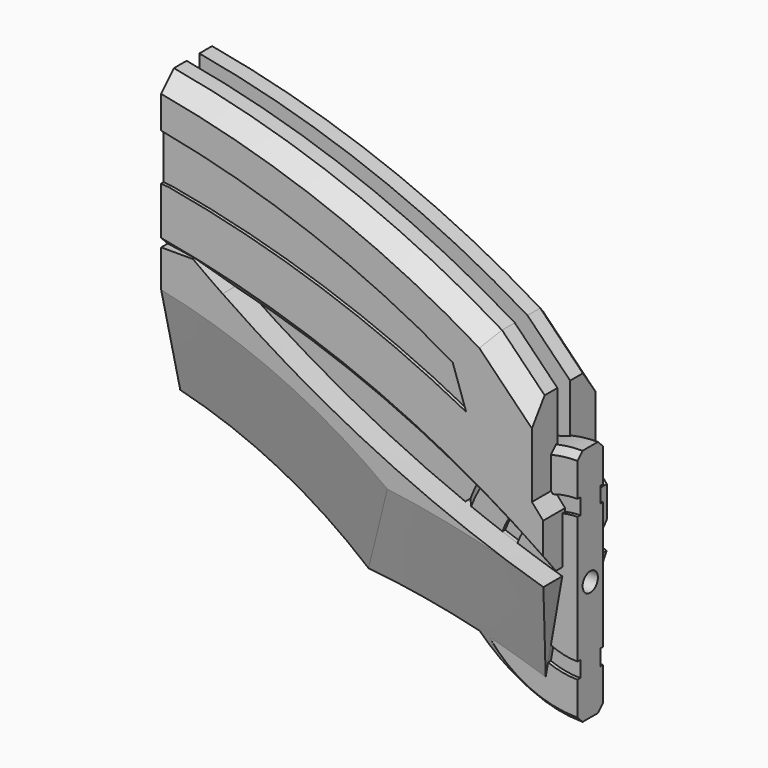
from build123d import *

# Parameters (mm, degrees)
F3_DEPTH     = 31.75
F5_DEPTH     = 6.35
F6_SIZE      = 12.7
F7_SIZE      = 12.7
F9_DEPTH     = 31.75
F11_DEPTH    = 12.7
F13_T2_ANGLE = 48.1784563201
F13_T4_ANGLE = 86.2150976381
F13_T6_ANGLE = 86.2150976381
F13_T8_ANGLE = 48.1784563201
F15_DEPTH    = 12.7
F16_SIZE     = 5.08
F18_DEPTH    = 2.54
F20_DEPTH    = 2.54
F21_R        = 7.62
F22_DEPTH    = 38.1
F24_DEPTH    = 2.794
F26_DEPTH    = 2.54
F27_R        = 10.16
F27_R_2      = 9.525
F28_DEPTH    = 76.2


# Not quite as in the source:
# - a fillet or chamfer that OpenCascade refuses, or shapes differently, is made with other operations: its cross-section is extruded or revolved along the edge and cut away or added
# - a feature of the source that left no trace in its solid (it failed there, or was rolled back) is left out
# - a feature names something its author has since deleted; it is built from what else it names


with BuildPart() as f3:
    # F2 (on Front) → F3 (new body, symmetric)
    with BuildSketch(Plane.XZ):
        with BuildLine():
            Line((37.9477068782, 57.15), (37.9477068782, -69.85))
            ThreePointArc((37.9477068782, -69.85), (197.3095607255, -116.6415507663), (342.7477068782, -196.85))
            Line((342.7477068782, -196.85), (342.7477068782, -156.4439684153))
            Line((342.7477068782, -156.4439684153), (333.764821291, -146.2200134993))
            Line((333.764821291, -146.2200134993), (333.764821291, -76.4565169811))
            Line((333.764821291, -76.4565169811), (299.7545793033, -41.7148783095))
            ThreePointArc((299.7545793033, -41.7148783095), (173.42869903, 19.8395158234), (37.9477068782, 57.15))
        make_face()
    extrude(amount=F3_DEPTH, both=True)

    # F4 (on Front) → F5 (cut, symmetric)
    with BuildSketch(Plane.XZ):
        with BuildLine():
            Line((37.9477068782, -48.4879799187), (37.9477068782, -69.85))
            ThreePointArc((37.9477068782, -69.85), (197.3095607255, -116.6415507663), (342.7477068782, -196.85))
            Line((342.7477068782, -196.85), (342.7477068782, -156.4439684153))
            Line((342.7477068782, -156.4439684153), (333.764821291, -146.2200134993))
            Line((333.764821291, -146.2200134993), (333.764821291, -76.4565169811))
            Line((333.764821291, -76.4565169811), (299.7545793033, -41.7148783095))
            ThreePointArc((299.7545793033, -41.7148783095), (173.42869903, 19.8395158234), (37.9477068782, 57.15))
            Line((37.9477068782, 57.15), (37.9477068782, 40.4159426689))
            ThreePointArc((37.9477068782, 40.4159426689), (174.1077804995, -9.1728518585), (291.3761138916, -94.3007096648))
            Line((291.3761138916, -94.3007096648), (297.9114055634, -145.1900005341))
            ThreePointArc((297.9114055634, -145.1900005341), (173.776538026, -81.1205697987), (37.9477068782, -48.4879799187))
        make_face()
    extrude(amount=F5_DEPTH, both=True, mode=Mode.SUBTRACT)

    # F6
    f6_edges = [f3.edges().sort_by_distance(p)[0] for p in [
        (173.428699, -31.75, 19.839516),
        (316.7597, -31.75, -59.085698),
        (316.7597, 31.75, -59.085698),
        (173.428699, 31.75, 19.839516),
    ]]
    chamfer(f6_edges, length=F6_SIZE)

    # F7
    f7_edges = [f3.edges().sort_by_distance(p)[0] for p in [
        (197.309561, -31.75, -116.641551),
        (197.309561, 31.75, -116.641551),
    ]]
    chamfer(f7_edges, length=F7_SIZE)

    # F8 (on Front) → F9 (join, symmetric)
    with BuildSketch(Plane.XZ):
        with BuildLine():
            ThreePointArc((86.9189181185, -80.2493599938), (62.5187399917, -74.647396796), (37.9477068782, -69.85))
            Line((37.9477068782, -69.85), (37.9477068782, -171.45))
            ThreePointArc((37.9477068782, -171.45), (117.3693749826, -201.1045334968), (188.127681613, -247.7998733521))
            ThreePointArc((188.127681613, -247.7998733521), (259.6802456544, -259.033648506), (329.51571574, -278.2423507795))
            Line((329.51571574, -278.2423507795), (342.7477068782, -203.2))
            ThreePointArc((342.7477068782, -203.2), (210.1366349445, -151.4972629597), (86.9189181185, -80.2493599938))
        make_face()
        with BuildLine():
            add(Edge.make_bspline(
                [(37.9477068782, -69.85), (37.9477068782, -67.7549506267), (37.9477068782, -65.6599012534), (37.9477068782, -63.5648518801)],
                knots=[0, 0, 0, 0, 0.4873412151, 0.4873412151, 0.4873412151, 0.4873412151], degree=3))
            ThreePointArc((37.9477068782, -69.85), (62.5187399917, -74.647396796), (86.9189181185, -80.2493599938))
            ThreePointArc((86.9189181185, -80.2493599938), (75.0688400161, -71.9981901024), (63.3477068782, -63.5648518801))
            Line((63.3477068782, -63.5648518801), (37.9477068782, -63.5648518801))
        make_face()
    extrude(amount=F9_DEPTH, both=True)

    # F10 (on Front) → F11 (cut, symmetric)
    with BuildSketch(Plane.XZ):
        with BuildLine():
            add(Edge.make_bspline(
                [(37.9477068782, -69.85), (37.9477068782, -67.7549506267), (37.9477068782, -65.6599012534), (37.9477068782, -63.5648518801)],
                knots=[0, 0, 0, 0, 0.4873412151, 0.4873412151, 0.4873412151, 0.4873412151], degree=3))
            Line((37.9477068782, -69.85), (37.9477068782, -171.45))
            ThreePointArc((37.9477068782, -171.45), (117.3693749826, -201.1045334968), (188.127681613, -247.7998733521))
            ThreePointArc((188.127681613, -247.7998733521), (259.6802456544, -259.033648506), (329.51571574, -278.2423507795))
            Line((329.51571574, -278.2423507795), (342.7477068782, -203.2))
            ThreePointArc((342.7477068782, -203.2), (197.1706361591, -145.1420264492), (63.3477068782, -63.5648518801))
            Line((63.3477068782, -63.5648518801), (37.9477068782, -63.5648518801))
        make_face()
    extrude(amount=F11_DEPTH, both=True, mode=Mode.SUBTRACT)

    # F13: chamfer of 76.2 x 19.05 on 4 edges, made by hand

    # F13_s1 → F13_t2 (revolve, cut)
    with BuildSketch(Plane(origin=(-60.6535291513, 0, -12.8240400006), x_dir=(0, 1, 0), z_dir=(-0.9783709739, 0, -0.2068580127))):
        Polygon((31.75, 174.9435450059), (12.7, 251.1435450059), (31.75, 251.1435450059), align=None)
    revolve(axis=Axis((124.3217755456, 31.75, -887.6969377111), (0, 1, 0)), revolution_arc=F13_T2_ANGLE, mode=Mode.SUBTRACT)

    # F13_s3 → F13_t4 (revolve, cut)
    with BuildSketch(Plane(origin=(-192.2531449662, 0, -55.7064857223), x_dir=(0, 1, 0), z_dir=(-0.9604918286, 0, -0.2783081876))):
        Polygon((12.7, 124.3402407106), (31.75, 48.1402407106), (31.75, 124.3402407106), align=None)
    revolve(axis=Axis((-53.0135938756, 31.75, -536.2473285656), (0, 1, 0)), revolution_arc=F13_T4_ANGLE, mode=Mode.SUBTRACT)

    # F13_s5 → F13_t6 (revolve, cut)
    with BuildSketch(Plane(origin=(-192.2531449662, 0, -55.7064857223), x_dir=(0, 1, 0), z_dir=(-0.9604918286, 0, -0.2783081876))):
        Polygon((-31.75, 48.1402407106), (-12.7, 124.3402407106), (-31.75, 124.3402407106), align=None)
    revolve(axis=Axis((-53.0135938756, -31.75, -536.2473285656), (0, 1, 0)), revolution_arc=F13_T6_ANGLE, mode=Mode.SUBTRACT)

    # F13_s7 → F13_t8 (revolve, cut)
    with BuildSketch(Plane(origin=(-60.6535291513, 0, -12.8240400006), x_dir=(0, 1, 0), z_dir=(-0.9783709739, 0, -0.2068580127))):
        Polygon((-31.75, 174.9435450059), (-12.7, 251.1435450059), (-31.75, 251.1435450059), align=None)
    revolve(axis=Axis((124.3217755456, -31.75, -887.6969377111), (0, 1, 0)), revolution_arc=F13_T8_ANGLE, mode=Mode.SUBTRACT)

    # F14 (on Front) → F15 (join, symmetric)
    with BuildSketch(Plane.XZ):
        with BuildLine():
            Line((354.91571574, -208.3923507795), (354.91571574, -113.1423507795))
            ThreePointArc((354.91571574, -113.1423507795), (259.66571574, -208.3923507795), (354.91571574, -303.6423507795))
            Line((354.91571574, -303.6423507795), (354.91571574, -208.3923507795))
        make_face()
    extrude(amount=F15_DEPTH, both=True)

    # F16
    f16_edges = [f3.edges().sort_by_distance(p)[0] for p in [
        (310.909323, -12.7, -292.867199),
        (270.087911, -12.7, -165.070232),
        (344.273637, -12.7, -113.738726),
        (344.273637, 12.7, -113.738726),
        (270.087911, 12.7, -165.070232),
        (310.909323, 12.7, -292.867199),
    ]]
    chamfer(f16_edges, length=F16_SIZE)

    # F17 (on face) → F18 (cut)
    with BuildSketch(Plane.XZ.offset(31.75)):
        with BuildLine():
            Line((37.9477068782, 18.4170784308), (37.9477068782, -18.7770907031))
            Line((37.9477068782, -18.7770907031), (44.5238578239, -19.4250085564))
            ThreePointArc((44.5238578239, -19.4250085564), (166.0160786587, -50.5371993601), (281.275870441, -99.9690568843))
            Line((281.275870441, -99.9690568843), (270.4956403873, -68.620350335))
            ThreePointArc((270.4956403873, -68.620350335), (157.9813255542, -15.0565404403), (37.9477068782, 18.4170784308))
        make_face()
    extrude(amount=-F18_DEPTH, mode=Mode.SUBTRACT)

    # F19 (on face) → F20 (cut)
    with BuildSketch(Plane(origin=(0, 31.75, 0), x_dir=(-1, 0, 0), z_dir=(0, 1, 0))):
        with BuildLine():
            ThreePointArc((-37.9477068782, 18.4170784308), (-157.9813255542, -15.0565404403), (-270.4956403873, -68.620350335))
            Line((-270.4956403873, -68.620350335), (-281.275870441, -99.9690568843))
            ThreePointArc((-281.275870441, -99.9690568843), (-166.0160786587, -50.5371993601), (-44.5238578239, -19.4250085564))
            Line((-44.5238578239, -19.4250085564), (-37.9477068782, -18.7770907031))
            Line((-37.9477068782, -18.7770907031), (-37.9477068782, 18.4170784308))
        make_face()
    extrude(amount=-F20_DEPTH, mode=Mode.SUBTRACT)

    # F21 (on face) → F22 (cut)
    with BuildSketch(Plane.YZ.offset(354.91571574)):
        with Locations((0, -208.3923507795)):
            Circle(F21_R)
    extrude(amount=-F22_DEPTH, mode=Mode.SUBTRACT)

    # F23 (on face) → F24 (cut)
    with BuildSketch(Plane.XZ.offset(12.7)):
        with BuildLine():
            ThreePointArc((331.4293971954, -267.3893239326), (342.9586633277, -270.7564341738), (354.91571574, -271.8923507795))
            Line((354.91571574, -271.8923507795), (354.91571574, -259.1923507795))
            ThreePointArc((354.91571574, -259.1923507795), (344.0535486893, -258.0174787588), (333.6938090461, -254.5472061718))
            Line((333.6938090461, -254.5472061718), (331.4293971954, -267.3893239326))
        make_face()
        with BuildLine():
            ThreePointArc((342.7477068782, -159.0711630369), (348.7869449547, -157.9634090034), (354.91571574, -157.5923507795))
            Line((354.91571574, -157.5923507795), (354.91571574, -144.8923507795))
            ThreePointArc((354.91571574, -144.8923507795), (344.9966028413, -145.6718501493), (335.3210156829, -147.991210644))
            Line((335.3210156829, -147.991210644), (342.7477068782, -156.4439684153))
            Line((342.7477068782, -156.4439684153), (342.7477068782, -159.0711630369))
        make_face()
        with BuildLine():
            ThreePointArc((303.5618689691, -171.0422179573), (298.710555552, -178.8418860075), (295.0352686554, -187.2598625929))
            ThreePointArc((295.0352686554, -187.2598625929), (301.0091143651, -189.413157651), (306.9974582895, -191.5257979926))
            ThreePointArc((306.9974582895, -191.5257979926), (310.1473048853, -184.3834068306), (314.3542442481, -177.8079261419))
            ThreePointArc((314.3542442481, -177.8079261419), (308.9721939736, -174.4025207151), (303.5618689691, -171.0422179573))
        make_face()
    extrude(amount=-F24_DEPTH, mode=Mode.SUBTRACT)

    # F25 (on face) → F26 (cut)
    with BuildSketch(Plane(origin=(0, 12.7, 0), x_dir=(-1, 0, 0), z_dir=(0, 1, 0))):
        with BuildLine():
            Line((-354.91571574, -259.1923507795), (-354.91571574, -271.8923507795))
            ThreePointArc((-354.91571574, -271.8923507795), (-342.9586633277, -270.7564341738), (-331.4293971954, -267.3893239326))
            Line((-331.4293971954, -267.3893239326), (-333.6938090461, -254.5472061718))
            ThreePointArc((-333.6938090461, -254.5472061718), (-344.0535486893, -258.0174787588), (-354.91571574, -259.1923507795))
        make_face()
        with BuildLine():
            ThreePointArc((-335.3210156829, -147.991210644), (-344.9966028413, -145.6718501493), (-354.91571574, -144.8923507795))
            Line((-354.91571574, -144.8923507795), (-354.91571574, -157.5923507795))
            ThreePointArc((-354.91571574, -157.5923507795), (-348.7869449547, -157.9634090034), (-342.7477068782, -159.0711630369))
            Line((-342.7477068782, -159.0711630369), (-342.7477068782, -156.4439684153))
            Line((-342.7477068782, -156.4439684153), (-335.3210156829, -147.991210644))
        make_face()
        with BuildLine():
            ThreePointArc((-295.0352686554, -187.2598625929), (-298.710555552, -178.8418860075), (-303.5618689691, -171.0422179573))
            ThreePointArc((-303.5618689691, -171.0422179573), (-308.9721939736, -174.4025207151), (-314.3542442481, -177.8079261419))
            ThreePointArc((-314.3542442481, -177.8079261419), (-310.1473048853, -184.3834068306), (-306.9974582895, -191.5257979926))
            ThreePointArc((-306.9974582895, -191.5257979926), (-301.0091143651, -189.413157651), (-295.0352686554, -187.2598625929))
        make_face()
    extrude(amount=-F26_DEPTH, mode=Mode.SUBTRACT)

    # F27 (on face) → F28 (cut)
    with BuildSketch(Plane(origin=(0, 0, 0), x_dir=(0, -1, 0), z_dir=(-1, 0, 0))):
        Circle(F27_R)
        Circle(F27_R_2, mode=Mode.SUBTRACT)
        Circle(F27_R_2)
    extrude(amount=-F28_DEPTH, mode=Mode.SUBTRACT)


solid = f3.part
